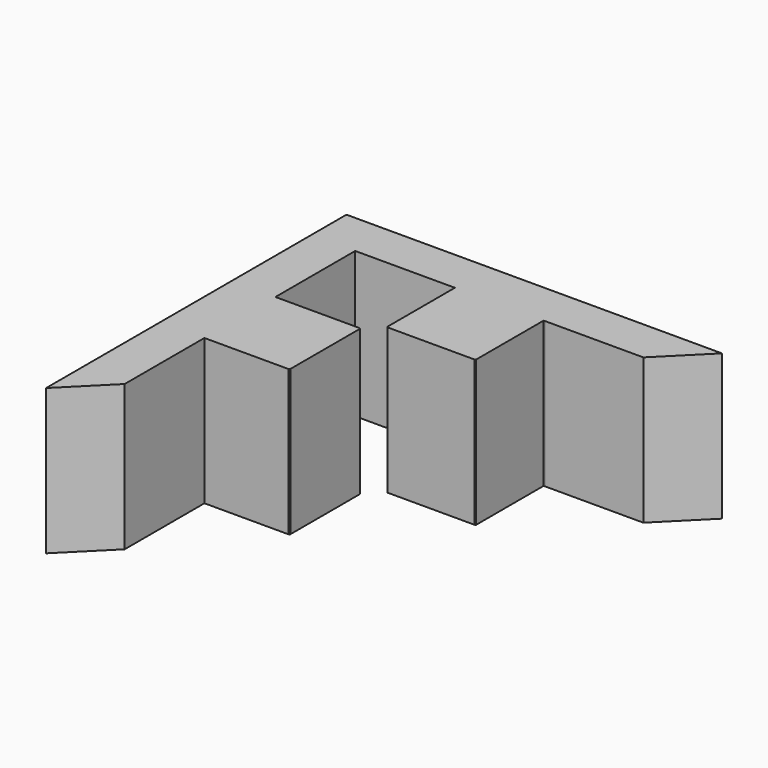
from build123d import *

# Parameters (mm, degrees)
F1_DEPTH = 10


# Not quite as in the source:
# - ends of sketch curves that miss each other by under 0.0002 mm in the source are joined


with BuildPart() as f1:
    # F0 (on Top) → F1 (new body)
    with BuildSketch(Plane.XY):
        Polygon((-9.9, 9.9), (-3.15, 9.9), (-3.05, 9.9), (-3.05, 8), (-3.05, 4.1106601718), (-2.9893398282, 4.05), (0, 4.05), (2.9893580109, 4.05), (3.0500181827, 4.1106601718), (3.0500181827, 7.9999861631), (3.0500181827, 9.8999861631), (3.1500181827, 9.9), (9.9000181827, 9.9), (12.9000181827, 12.9), (1.81827e-05, 12.9), (-12.9, 12.9), (-12.9, 0), (-12.9, -12.9000181827), (-9.9, -9.9000181827), (-9.9, -3.1500181827), (-9.9, -3.0500181827), (-7.999823753, -3.0500181827), (-4.1106601718, -3.0500181827), (-4.05, -2.9893580109), (-4.05, -3.36409e-05), (-4.05, 2.9893398282), (-4.1106601718, 3.05), (-8, 3.05), (-9.9, 3.05), (-9.9, 3.15), align=None)
    extrude(amount=F1_DEPTH)


solid = f1.part
